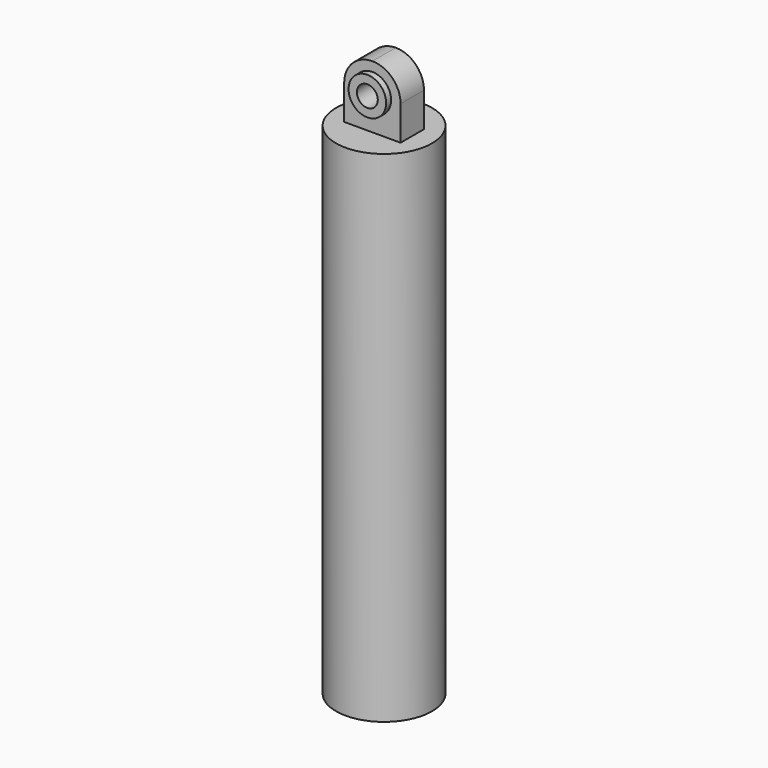
from build123d import *

# Parameters (mm, degrees)
F0_R      = 29.21
F1_DEPTH  = 304.165
F2_W      = 34.29
F2_H      = 17.78
F3_DEPTH  = 38.1
F4_R      = 17.14499
F5_R      = 11.43
F6_DEPTH  = 3.81
F7_R      = 11.43
F8_DEPTH  = 3.81
F9_R      = 6.35
F10_DEPTH = 38.1


# Not quite as in the source:
# - a fillet or chamfer is up to 0.001 mm smaller than in the source, because OpenCascade refuses the exact size


with BuildPart() as f1:
    # F0 (on Top) → F1 (new body)
    with BuildSketch(Plane.XY):
        Circle(F0_R)
    extrude(amount=F1_DEPTH)

    # F2 (on face) → F3 (join)
    with BuildSketch(Plane.XY.offset(304.165)):
        Rectangle(F2_W, F2_H)
    extrude(amount=F3_DEPTH)

    # F4 (radius 17.145 in the source; OpenCascade refuses exactly that, so slightly less here)
    f4_edges = [f1.edges().sort_by_distance(p)[0] for p in [
        (17.145, 0, 342.265),
        (-17.145, 0, 342.265),
    ]]
    fillet(f4_edges, radius=F4_R)

    # F5 (on face) → F6 (join)
    with BuildSketch(Plane(origin=(0, 8.89, 0), x_dir=(-1, 0, 0), z_dir=(0, 1, 0))):
        with Locations((0, 325.12)):
            Circle(F5_R)
    extrude(amount=F6_DEPTH)

    # F7 (on face) → F8 (join)
    with BuildSketch(Plane.XZ.offset(8.89)):
        with Locations((0, 325.12)):
            Circle(F7_R)
    extrude(amount=F8_DEPTH)

    # F9 (on face) → F10 (cut)
    with BuildSketch(Plane.XZ.offset(12.7)):
        with Locations((0, 325.12)):
            Circle(F9_R)
    extrude(amount=-F10_DEPTH, mode=Mode.SUBTRACT)


solid = f1.part
